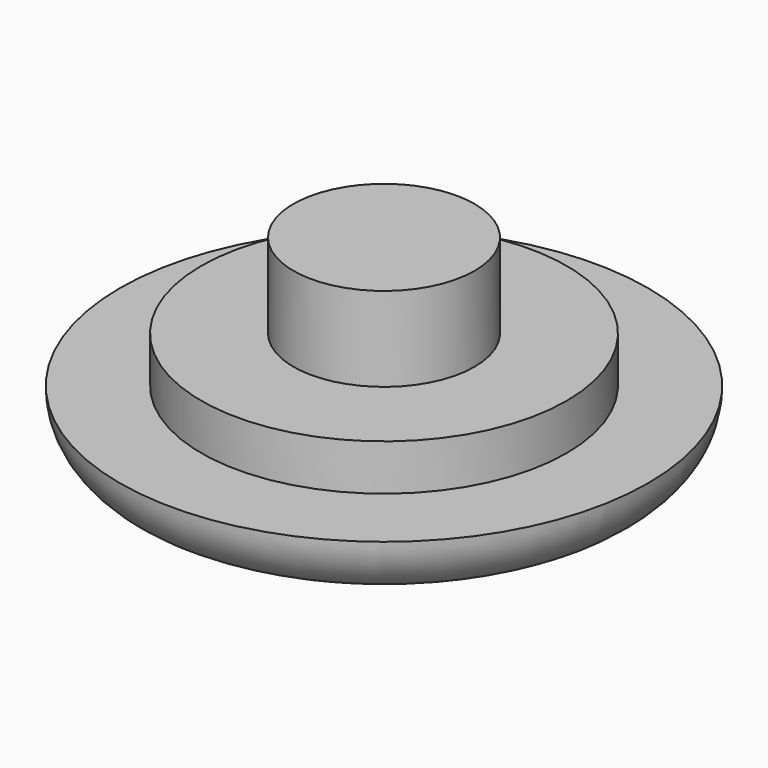
from build123d import *

# Parameters (mm, degrees)
F0_R     = 8.6
F0_R_2   = 5.95
F1_DEPTH = 2
F0_R_3   = 2.95
F2_DEPTH = 3.5
F3_DEPTH = 6.25
F4_R     = 1.99999


# Not quite as in the source:
# - a fillet or chamfer is up to 0.001 mm smaller than in the source, because OpenCascade refuses the exact size
# - a feature names something its author has since deleted; it is built from what else it names


with BuildPart() as f1:
    # F0 (on Top) → F1 (new body)
    with BuildSketch(Plane.XY):
        with Locations((-45.6172116101, 18.5634717345)):
            Circle(F0_R)
        with Locations((-45.6172116101, 18.5634717345)):
            Circle(F0_R_2, mode=Mode.SUBTRACT)
    extrude(amount=F1_DEPTH)

    # F0 (on Top) → F2 (join)
    with BuildSketch(Plane.XY):
        with Locations((-45.6172116101, 18.5634717345)):
            Circle(F0_R_2)
        with Locations((-45.6172116101, 18.5634717345)):
            Circle(F0_R_3, mode=Mode.SUBTRACT)
    extrude(amount=F2_DEPTH)

    # F0 (on Top) → F3 (join)
    with BuildSketch(Plane.XY):
        with Locations((-45.6172116101, 18.5634717345)):
            Circle(F0_R_3)
    extrude(amount=F3_DEPTH)

    # F4 (radius 2 in the source; OpenCascade refuses exactly that, so slightly less here)
    f4_edges = [f1.edges().sort_by_distance(p)[0] for p in [
        (-54.217212, 18.563472, 0),
    ]]
    fillet(f4_edges, radius=F4_R)


solid = f1.part
